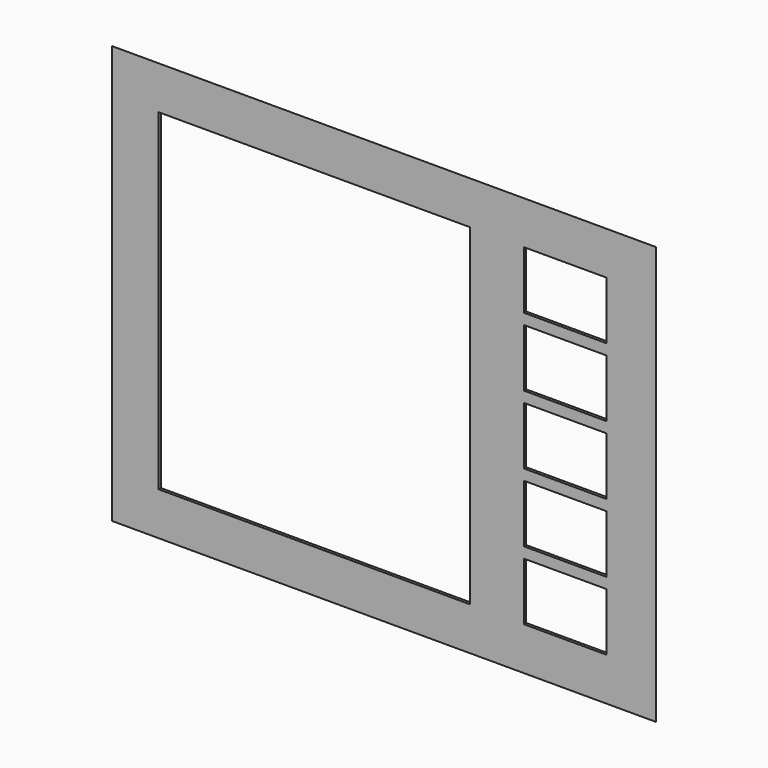
from build123d import *

# Parameters (mm, degrees)
F0_W     = 115
F0_H     = 80.54
F0_W_2   = 434
F0_H_2   = 462.7
F1_DEPTH = 4
F2_SIZE  = 3.99999


# Not quite as in the source:
# - a fillet or chamfer is up to 0.001 mm smaller than in the source, because OpenCascade refuses the exact size


with BuildPart() as f1:
    # F0 (on Front) → F1 (new body)
    with BuildSketch(Plane.XZ):
        Polygon((0, 582.7), (0, 0), (509, 0), (559, 0), (758, 0), (758, 582.7), (559, 582.7), (509, 582.7), align=None)
        with Locations((631.5, 100.27)):
            Rectangle(F0_W, F0_H, mode=Mode.SUBTRACT)
        with Locations((631.5, 195.81)):
            Rectangle(F0_W, F0_H, mode=Mode.SUBTRACT)
        with Locations((282, 291.35)):
            Rectangle(F0_W_2, F0_H_2, mode=Mode.SUBTRACT)
        with Locations((631.5, 291.35)):
            Rectangle(F0_W, F0_H, mode=Mode.SUBTRACT)
        with Locations((631.5, 386.89)):
            Rectangle(F0_W, F0_H, mode=Mode.SUBTRACT)
        with Locations((631.5, 482.43)):
            Rectangle(F0_W, F0_H, mode=Mode.SUBTRACT)
    extrude(amount=F1_DEPTH)

    # F2 (size 4 in the source; OpenCascade refuses exactly that, so slightly less here)
    f2_edges = [f1.edges().sort_by_distance(p)[0] for p in [
        (379, 0, 0),
        (758, 0, 291.35),
        (0, 0, 291.35),
        (379, 0, 582.7),
    ]]
    chamfer(f2_edges, length=F2_SIZE)


solid = f1.part
